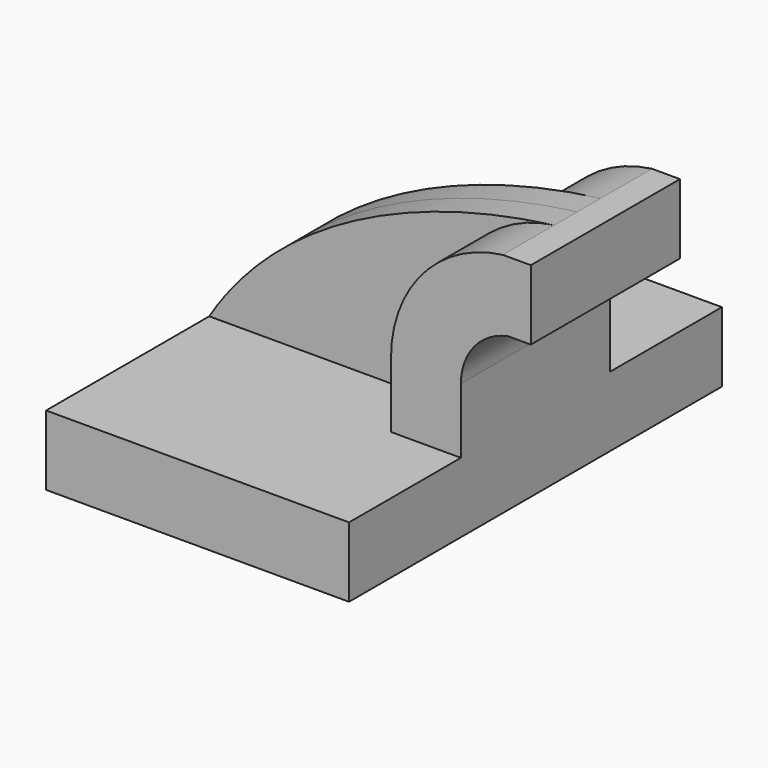
from build123d import *

# Parameters (mm, degrees)
F1_DEPTH = 63.5
F2_DEPTH = 25.4
F3_DEPTH = 7.9375


with BuildPart() as f1:
    # F0 (on Front) → F1 (new body, symmetric)
    with BuildSketch(Plane.XZ):
        Polygon((-41.275, -9.525), (41.275, -9.525), (41.275, 9.525), (22.225, 9.525), (-41.275, 9.525), align=None)
    extrude(amount=F1_DEPTH, both=True)

    # F0 (on Front) → F2 (join, symmetric)
    with BuildSketch(Plane.XZ):
        with BuildLine():
            Line((22.225, 9.525), (41.275, 9.525))
            Line((41.275, 9.525), (41.275, 27.2855908291))
            ThreePointArc((41.275, 27.2855908291), (44.9109862911, 37.3960887611), (54.1533834246, 42.8752))
            Line((54.1533834246, 42.8752), (60.325, 42.8752))
            Line((60.325, 42.8752), (60.325, 61.9252))
            Line((60.325, 61.9252), (52.6943180668, 61.9252))
            ThreePointArc((52.6943180668, 61.9252), (30.926248204, 50.3522435282), (22.225, 27.2855908291))
            Line((22.225, 27.2855908291), (22.225, 9.525))
        make_face()
    extrude(amount=F2_DEPTH, both=True)

    # F0 (on Front) → F3 (join, symmetric)
    with BuildSketch(Plane.XZ):
        with BuildLine():
            add(Edge.make_bspline(
                [(52.6943180668, 61.9252), (15.7995279878, 57.229410857), (-21.768245846, 41.0787798464), (-41.275, 9.525)],
                knots=[0, 0, 0, 0, 107.5918849076, 107.5918849076, 107.5918849076, 107.5918849076], degree=3))
            Line((-41.275, 9.525), (22.225, 9.525))
            Line((22.225, 9.525), (22.225, 27.2855908291))
            ThreePointArc((22.225, 27.2855908291), (30.926248204, 50.3522435282), (52.6943180668, 61.9252))
        make_face()
    extrude(amount=F3_DEPTH, both=True)


solid = f1.part
